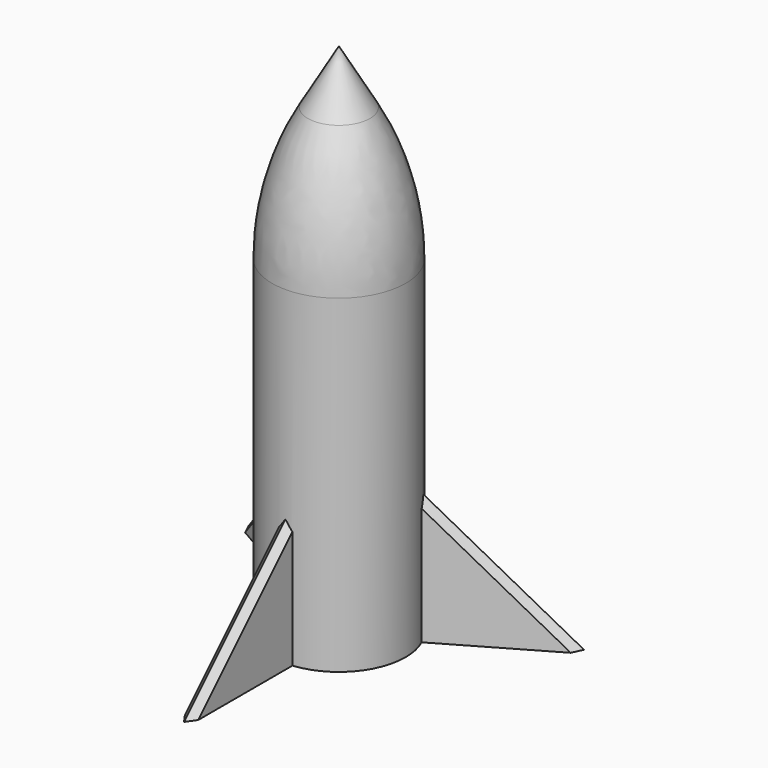
from build123d import *

# Parameters (mm, degrees)
F0_R      = 12.7
F1_DEPTH  = 76.2
F1_FACE_R = 12.7
F2_DEPTH  = 25.4
F2_TAPER  = 30
F3_R      = 50.8
F4_T      = -2.54
F6_DEPTH  = 1.27
F7_SIZE   = 1.2699
F8_COUNT  = 3


# Not quite as in the source:
# - a fillet or chamfer is up to 0.001 mm smaller than in the source, because OpenCascade refuses the exact size


with BuildPart() as f1:
    # F0 (on Top) → F1 (new body)
    with BuildSketch(Plane.XY):
        Circle(F0_R)
    extrude(amount=F1_DEPTH)

    # F1_face (on face) → F2 (join)
    with BuildSketch(Plane.XY.offset(76.2)):
        Circle(F1_FACE_R)
    extrude(amount=F2_DEPTH, taper=F2_TAPER)

    # F3
    f3_edges = [f1.edges().sort_by_distance(p)[0] for p in [
        (-12.7, 0, 76.2),
    ]]
    fillet(f3_edges, radius=F3_R)

    # F4
    f4_openings = [f1.faces().sort_by_distance(p)[0] for p in [
        (0, 0, 0),
    ]]
    offset(amount=F4_T, openings=f4_openings)

    # F5 (on Right) → F6 (join, symmetric)
    with BuildSketch(Plane.YZ):
        Polygon((-36.83, 0), (-11.43, 0), (-11.43, 25.4), align=None)
    extrude(amount=F6_DEPTH, both=True)

    # F7 (size 1.27 in the source; OpenCascade refuses exactly that, so slightly less here)
    f7_edges = [f1.edges().sort_by_distance(p)[0] for p in [
        (1.27, -24.73317, 12.09683),
        (-1.27, -24.73317, 12.09683),
    ]]
    chamfer(f7_edges, length=F7_SIZE)

    # F8: F1 ×3 about axis
    f8_axis = Axis((0, 0, 0), (0, 0, 1))


with BuildPart() as f1_1:
    add(f1.part)
    for i in range(1, F8_COUNT):
        add(f1.part.rotate(f8_axis, i * 360 / F8_COUNT))


solid = f1_1.part
